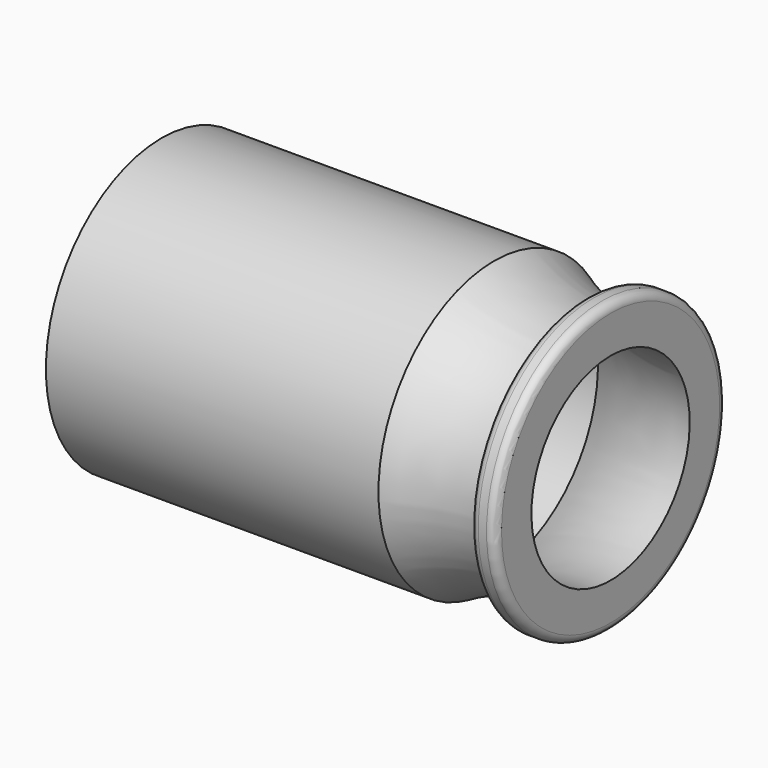
from build123d import *

# Parameters (mm, degrees)
F2_R = 1
F3_R = 0.6


# Not quite as in the source:
# - a feature names something its author has since deleted; it is built from what else it names


with BuildPart() as f1:
    # F0 (on Front) → F1 (revolve)
    with BuildSketch(Plane.XZ):
        with BuildLine():
            Line((40, 17.4), (11.5, 17.4))
            Line((11.5, 17.4), (0, 17.4))
            Line((0, 17.4), (0, 15.6))
            Line((0, 15.6), (40, 15.6))
            ThreePointArc((40, 15.6), (46.7596616101, 12.8406114977), (54, 11.9))
            Line((54, 11.9), (54, 17.4))
            Line((54, 17.4), (51, 17.4))
            Line((51, 17.4), (51, 14.4))
            ThreePointArc((51, 14.4), (45.2991228745, 15.1634505398), (40, 17.4))
        make_face()
    revolve(axis=Axis((27, 0, 0), (1, 0, 0)))

    # F2
    f2_edges = [f1.edges().sort_by_distance(p)[0] for p in [
        (54, 0, -17.4),
        (51, 0, -17.4),
    ]]
    fillet(f2_edges, radius=F2_R)

    # F3
    f3_edges = [f1.edges().sort_by_distance(p)[0] for p in [
        (0, 0, -15.6),
    ]]
    fillet(f3_edges, radius=F3_R)


solid = f1.part
